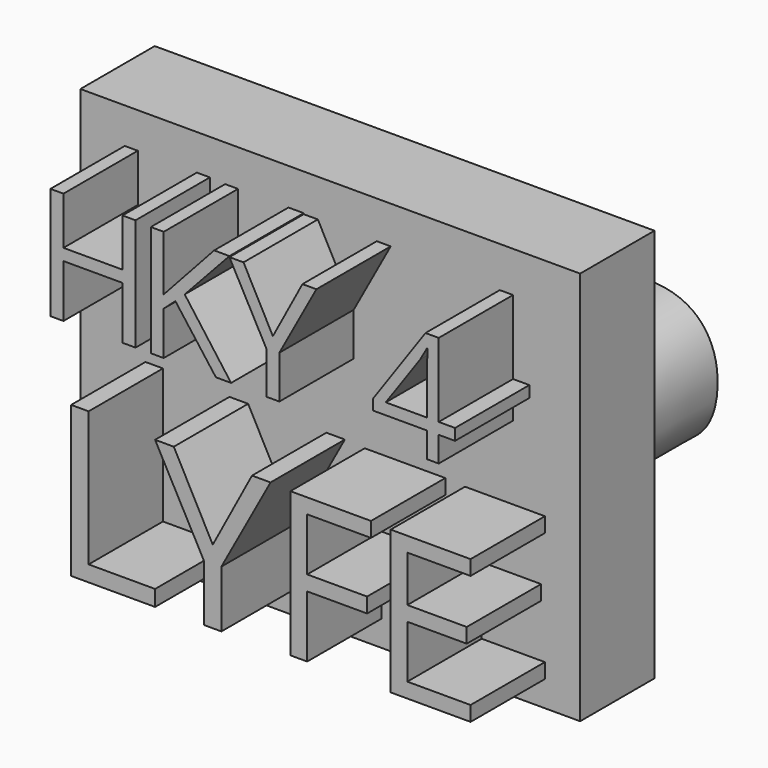
from build123d import *

# Parameters (mm, degrees)
F0_W          = 136.6110444069
F0_H          = 107.7354475856
F1_DEPTH      = 25.4
F2_TEXT_SIZE  = 42.9226900451
F3_DEPTH      = 25.4
F4_TEXT_SIZE  = 42.5594120694
F5_DEPTH      = 25.4
F6_TEXT_SIZE  = 42.4625388766
F7_DEPTH      = 25.4
F8_TEXT_SIZE  = 42.1327021387
F9_DEPTH      = 25.4
F10_TEXT_SIZE = 57.6691365697
F11_DEPTH     = 25.4
F12_TEXT_SIZE = 56.3524896279
F13_DEPTH     = 25.4
F14_TEXT_SIZE = 55.348890242
F15_DEPTH     = 25.4
F16_TEXT_SIZE = 54.8804426032
F17_DEPTH     = 25.4
F18_TEXT_SIZE = 50.0173730841
F19_DEPTH     = 25.4
F20_TEXT_SIZE = 45.6684326214
F21_DEPTH     = 25.4
F22_TEXT_SIZE = 45.5559839288
F23_DEPTH     = 25.4
F24_TEXT_SIZE = 41.0793840678
F25_DEPTH     = 25.4


# Not quite as in the source:
# - Text() gives the source's letters only with a copy of the font that has no kerning and outlines rounded to 1/6400 em; it was checked with that copy


with BuildPart() as f1:
    # F0 (on Front) → F1 (new body)
    with BuildSketch(Plane.XZ):
        with Locations((-2.4629384279, -5.2130073309)):
            Rectangle(F0_W, F0_H)
    extrude(amount=F1_DEPTH)

    # F2 (on face) → F3 (join)
    with BuildSketch(Plane.XZ.offset(25.4)):
        with Locations((-62.8514587879, 8.2474770024)):
            Text('H', F2_TEXT_SIZE, font='Open Sans', text_align=(TextAlign.LEFT, TextAlign.BOTTOM))
    extrude(amount=F3_DEPTH)

    # F4 (on face) → F5 (join)
    with BuildSketch(Plane.XZ.offset(25.4)):
        with Locations((-35.3742304887, 8.2474770024)):
            Text('K', F4_TEXT_SIZE, font='Open Sans', text_align=(TextAlign.LEFT, TextAlign.BOTTOM))
    extrude(amount=F5_DEPTH)

    # F6 (on face) → F7 (join)
    with BuildSketch(Plane.XZ.offset(25.4)):
        with Locations((-9.7122349925, 8.057879284)):
            Text('Y', F6_TEXT_SIZE, font='Open Sans', text_align=(TextAlign.LEFT, TextAlign.BOTTOM))
    extrude(amount=F7_DEPTH)

    # F8 (on face) → F9 (join)
    with BuildSketch(Plane.XZ.offset(25.4)):
        with Locations((28.7239681929, 7.299490273)):
            Text('4', F8_TEXT_SIZE, font='Open Sans', text_align=(TextAlign.LEFT, TextAlign.BOTTOM))
    extrude(amount=F9_DEPTH)

    # F10 (on face) → F11 (join)
    with BuildSketch(Plane.XZ.offset(25.4)):
        with Locations((-58.6396698272, -52.4236150086)):
            Text('L', F10_TEXT_SIZE, font='Open Sans', text_align=(TextAlign.LEFT, TextAlign.BOTTOM))
    extrude(amount=F11_DEPTH)

    # F12 (on face) → F13 (join)
    with BuildSketch(Plane.XZ.offset(25.4)):
        with Locations((-30.0303716071, -52.4236150086)):
            Text('Y', F12_TEXT_SIZE, font='Open Sans', text_align=(TextAlign.LEFT, TextAlign.BOTTOM))
    extrude(amount=F13_DEPTH)

    # F14 (on face) → F15 (join)
    with BuildSketch(Plane.XZ.offset(25.4)):
        with Locations((1.5270225845, -52.0444214344)):
            Text('F', F14_TEXT_SIZE, font='Open Sans', text_align=(TextAlign.LEFT, TextAlign.BOTTOM))
    extrude(amount=F15_DEPTH)

    # F16 (on face) → F17 (join)
    with BuildSketch(Plane.XZ.offset(25.4)):
        with Locations((28.985261103, -52.0444214344)):
            Text('E', F16_TEXT_SIZE, font='Open Sans', text_align=(TextAlign.LEFT, TextAlign.BOTTOM))
    extrude(amount=F17_DEPTH)

    # F18 (on face) → F19 (join)
    with BuildSketch(Plane(origin=(0, 0, 0), x_dir=(-1, 0, 0), z_dir=(0, 1, 0))):
        with Locations((-65.8425837755, -16.9579970585)):
            Text('G', F18_TEXT_SIZE, font='Open Sans', text_align=(TextAlign.LEFT, TextAlign.BOTTOM))
    extrude(amount=F19_DEPTH)

    # F20 (on face) → F21 (join)
    with BuildSketch(Plane(origin=(0, 0, 0), x_dir=(-1, 0, 0), z_dir=(0, 1, 0))):
        with Locations((-30.0511494279, -15.8313624561)):
            Text('A', F20_TEXT_SIZE, font='Open Sans', text_align=(TextAlign.LEFT, TextAlign.BOTTOM))
    extrude(amount=F21_DEPTH)

    # F22 (on face) → F23 (join)
    with BuildSketch(Plane(origin=(0, 0, 0), x_dir=(-1, 0, 0), z_dir=(0, 1, 0))):
        with Locations((2.3699644953, -15.4521679506)):
            Text('B', F22_TEXT_SIZE, font='Open Sans', text_align=(TextAlign.LEFT, TextAlign.BOTTOM))
    extrude(amount=F23_DEPTH)

    # F24 (on face) → F25 (join)
    with BuildSketch(Plane(origin=(0, 0, 0), x_dir=(-1, 0, 0), z_dir=(0, 1, 0))):
        with Locations((32.7055081725, -12.9874050617)):
            Text('Y', F24_TEXT_SIZE, font='Open Sans', text_align=(TextAlign.LEFT, TextAlign.BOTTOM))
    extrude(amount=F25_DEPTH)


solid = f1.part
